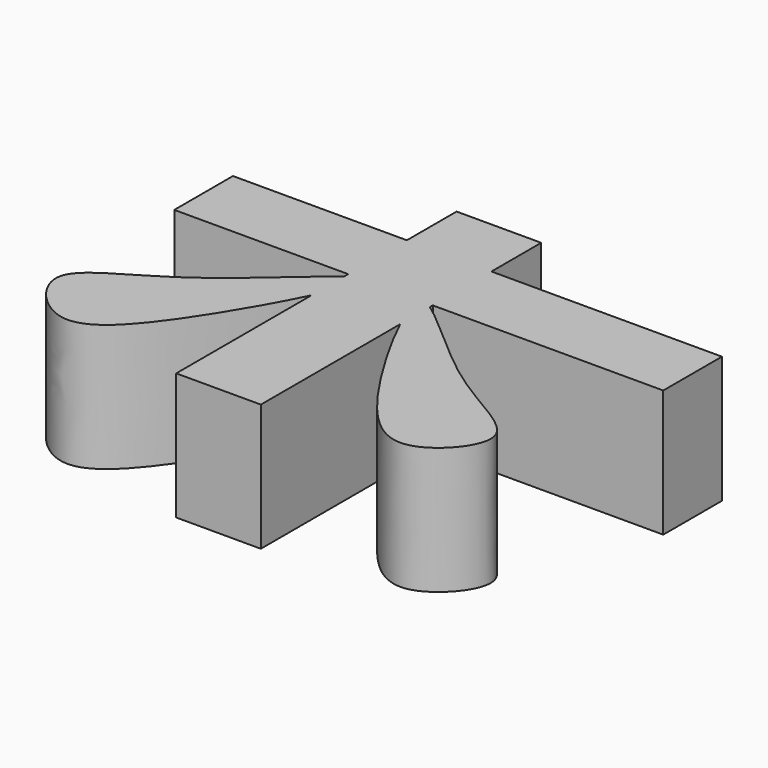
from build123d import *

# Parameters (mm, degrees)
F0_W     = 5.3317777347
F0_H     = 3.9184228517
F0_W_2   = 10.9595907852
F0_H_2   = 4.6226084232
F0_W_3   = 14.5260256249
F1_DEPTH = 8


# Not quite as in the source:
# - a feature names something its author has since deleted; it is built from what else it names


with BuildPart() as f1:
    # F0 (on Top) → F1 (new body)
    with BuildSketch(Plane.XY):
        with BuildLine():
            Line((2.5887365919, 22.509759292), (-2.7430411428, 22.509759292))
            Line((-2.7430411428, 22.509759292), (-2.7430411428, 17.8871508688))
            Line((-2.7430411428, 17.8871508688), (-2.1714857529, 17.8871508688))
            add(Edge.make_bspline(
                [(-1.8442005385, 17.8871508688), (-1.9073601168, 17.9527169942), (-2.0187846445, 17.9485893157), (-2.1714857529, 17.8871508688)],
                knots=[0, 0, 0, 0, 0.0293672898, 0.0293672898, 0.0293672898, 0.0293672898], degree=3))
            Line((-1.8442005385, 17.8871508688), (1.8442005385, 17.8871508688))
            add(Edge.make_bspline(
                [(1.8442005385, 17.8871508688), (1.9073601168, 17.9527169942), (2.0187846445, 17.9485893157), (2.1714857529, 17.8871508688)],
                knots=[0, 0, 0, 0, 0.0293672898, 0.0293672898, 0.0293672898, 0.0293672898], degree=3))
            Line((2.1714857529, 17.8871508688), (2.5887365919, 17.8871508688))
            Line((2.5887365919, 17.8871508688), (2.5887365919, 22.509759292))
        make_face()
        with Locations((-0.0771522755, 24.4689707179)):
            Rectangle(F0_W, F0_H)
        with Locations((-8.2228365354, 20.1984550804)):
            Rectangle(F0_W_2, F0_H_2)
        with BuildLine():
            add(Edge.make_bspline(
                [(2.1714857529, 17.8871508688), (2.287691695, 17.8403960503), (2.4278019357, 17.7604511347), (2.5887365919, 17.652773519)],
                knots=[0.0293672898, 0.0293672898, 0.0293672898, 0.0293672898, 0.051715874, 0.051715874, 0.051715874, 0.051715874], degree=3))
            Line((2.1714857529, 17.8871508688), (1.8442005385, 17.8871508688))
            add(Edge.make_bspline(
                [(2.5887365919, 15.3246397381), (1.9645139549, 16.6601739446), (1.6320309917, 17.6668971006), (1.8442005385, 17.8871508688)],
                knots=[0.9013475906, 0.9013475906, 0.9013475906, 0.9013475906, 1, 1, 1, 1], degree=3))
            Line((2.5887365919, 15.3246397381), (2.5887365919, 17.652773519))
        make_face()
        with Locations((9.8517494043, 20.1984550804)):
            Rectangle(F0_W_3, F0_H_2)
        with BuildLine():
            Line((-2.7430411428, 15.0000628183), (-2.7430411428, 17.5457150476))
            add(Edge.make_bspline(
                [(-2.7430411428, 17.5457150476), (-4.0179544262, 16.6326728497), (-9.1765243527, 11.5359259625), (-15.5039563603, 9.4932798244), (-10.823733112, 4.1142195469), (-7.1214858799, 7.1819415818), (-3.6930140846, 13.0335276913), (-2.7430411428, 15.0000628183)],
                knots=[0.0585891222, 0.0585891222, 0.0585891222, 0.0585891222, 0.2228561947, 0.4193627461, 0.5728239375, 0.7534217718, 0.8935035971, 0.8935035971, 0.8935035971, 0.8935035971], degree=3))
        make_face()
        with BuildLine():
            add(Edge.make_bspline(
                [(2.5887365919, 17.652773519), (3.8211371956, 16.8282030892), (9.0919520737, 11.5632279135), (15.5039563603, 9.4932798244), (10.823733112, 4.1142195469), (7.0602374067, 7.2326927282), (3.5247364856, 13.3220531586), (2.5887365919, 15.3246397381)],
                knots=[0.051715874, 0.051715874, 0.051715874, 0.051715874, 0.2228561947, 0.4193627461, 0.5728239375, 0.7534217718, 0.9013475906, 0.9013475906, 0.9013475906, 0.9013475906], degree=3))
            Line((2.5887365919, 17.652773519), (2.5887365919, 15.3246397381))
        make_face()
        with BuildLine():
            Line((-1.8442005385, 17.8871508688), (-2.1714857529, 17.8871508688))
            add(Edge.make_bspline(
                [(-2.1714857529, 17.8871508688), (-2.323430526, 17.8260167292), (-2.516244003, 17.7081381407), (-2.7430411428, 17.5457150476)],
                knots=[0.0293672898, 0.0293672898, 0.0293672898, 0.0293672898, 0.0585891222, 0.0585891222, 0.0585891222, 0.0585891222], degree=3))
            Line((-2.7430411428, 17.5457150476), (-2.7430411428, 15.0000628183))
            add(Edge.make_bspline(
                [(-2.7430411428, 15.0000628183), (-2.0208296717, 16.4951098503), (-1.615161089, 17.64938441), (-1.8442005385, 17.8871508688)],
                knots=[0.8935035971, 0.8935035971, 0.8935035971, 0.8935035971, 1, 1, 1, 1], degree=3))
        make_face()
        with BuildLine():
            Line((1.8442005385, 17.8871508688), (-1.8442005385, 17.8871508688))
            add(Edge.make_bspline(
                [(-2.7430411428, 15.0000628183), (-2.0208296717, 16.4951098503), (-1.615161089, 17.64938441), (-1.8442005385, 17.8871508688)],
                knots=[0.8935035971, 0.8935035971, 0.8935035971, 0.8935035971, 1, 1, 1, 1], degree=3))
            Line((-2.7430411428, 15.0000628183), (-2.7430411428, 4.3423823081))
            Line((-2.7430411428, 4.3423823081), (2.5887365919, 4.3423823081))
            Line((2.5887365919, 4.3423823081), (2.5887365919, 15.3246397381))
            add(Edge.make_bspline(
                [(2.5887365919, 15.3246397381), (1.9645139549, 16.6601739446), (1.6320309917, 17.6668971006), (1.8442005385, 17.8871508688)],
                knots=[0.9013475906, 0.9013475906, 0.9013475906, 0.9013475906, 1, 1, 1, 1], degree=3))
        make_face()
        with BuildLine():
            Line((2.5887365919, 17.652773519), (2.5887365919, 17.8871508688))
            Line((2.5887365919, 17.8871508688), (2.1714857529, 17.8871508688))
            add(Edge.make_bspline(
                [(2.1714857529, 17.8871508688), (2.287691695, 17.8403960503), (2.4278019357, 17.7604511347), (2.5887365919, 17.652773519)],
                knots=[0.0293672898, 0.0293672898, 0.0293672898, 0.0293672898, 0.051715874, 0.051715874, 0.051715874, 0.051715874], degree=3))
        make_face()
        with BuildLine():
            Line((-2.1714857529, 17.8871508688), (-2.7430411428, 17.8871508688))
            Line((-2.7430411428, 17.8871508688), (-2.7430411428, 17.5457150476))
            add(Edge.make_bspline(
                [(-2.1714857529, 17.8871508688), (-2.323430526, 17.8260167292), (-2.516244003, 17.7081381407), (-2.7430411428, 17.5457150476)],
                knots=[0.0293672898, 0.0293672898, 0.0293672898, 0.0293672898, 0.0585891222, 0.0585891222, 0.0585891222, 0.0585891222], degree=3))
        make_face()
        with BuildLine():
            add(Edge.make_bspline(
                [(-1.8442005385, 17.8871508688), (-1.9073601168, 17.9527169942), (-2.0187846445, 17.9485893157), (-2.1714857529, 17.8871508688)],
                knots=[0, 0, 0, 0, 0.0293672898, 0.0293672898, 0.0293672898, 0.0293672898], degree=3))
            Line((-2.1714857529, 17.8871508688), (-1.8442005385, 17.8871508688))
        make_face()
        with BuildLine():
            Line((1.8442005385, 17.8871508688), (2.1714857529, 17.8871508688))
            add(Edge.make_bspline(
                [(1.8442005385, 17.8871508688), (1.9073601168, 17.9527169942), (2.0187846445, 17.9485893157), (2.1714857529, 17.8871508688)],
                knots=[0, 0, 0, 0, 0.0293672898, 0.0293672898, 0.0293672898, 0.0293672898], degree=3))
        make_face()
    extrude(amount=F1_DEPTH)


solid = f1.part
